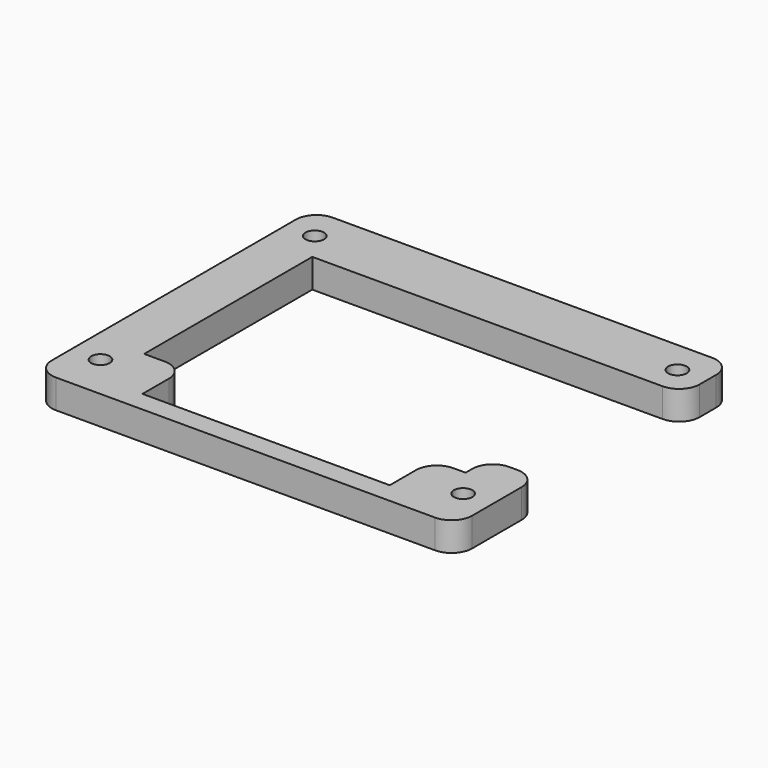
from build123d import *

# Parameters (mm, degrees)
F0_W     = 102
F0_H     = 84
F0_R     = 2.25
F0_W_2   = 78
F0_H_2   = 51
F1_DEPTH = 15
F3_DEPTH = 4
F4_W     = 12
F4_H     = 44
F4_W_2   = 60
F4_H_2   = 13
F5_DEPTH = 15.001
F6_W     = 102
F6_H     = 84
F7_DEPTH = 8
F8_R     = 5


with BuildPart() as f1:
    # F0 (on Top) → F1 (new body)
    with BuildSketch(Plane.XY):
        with Locations((0, -1.5)):
            Rectangle(F0_W, F0_H)
        with Locations((-44, -32.5)):
            Circle(F0_R, mode=Mode.SUBTRACT)
        with Locations((44, -32.5)):
            Circle(F0_R, mode=Mode.SUBTRACT)
        with Locations((-44, 32.5)):
            Circle(F0_R, mode=Mode.SUBTRACT)
        Rectangle(F0_W_2, F0_H_2, mode=Mode.SUBTRACT)
        with Locations((44, 32.5)):
            Circle(F0_R, mode=Mode.SUBTRACT)
    extrude(amount=F1_DEPTH)

    # F2 (on face) → F3 (cut)
    with BuildSketch(Plane(origin=(0, 0, 0), x_dir=(1, 0, 0), z_dir=(0, 0, -1))):
        Polygon((-41.075, 30.8112504626), (-41.075, 34.1887495374), (-44, 35.8774990748), (-46.925, 34.1887495374), (-46.925, 30.8112504626), (-44, 29.1225009252), align=None)
        Polygon((41.075, 34.1887495374), (41.075, 30.8112504626), (44, 29.1225009252), (46.925, 30.8112504626), (46.925, 34.1887495374), (44, 35.8774990748), align=None)
        Polygon((41.075, -30.8112504626), (41.075, -34.1887495374), (44, -35.8774990748), (46.925, -34.1887495374), (46.925, -30.8112504626), (44, -29.1225009252), align=None)
        Polygon((-41.075, -34.1887495374), (-41.075, -30.8112504626), (-44, -29.1225009252), (-46.925, -30.8112504626), (-46.925, -34.1887495374), (-44, -35.8774990748), align=None)
    extrude(amount=-F3_DEPTH, mode=Mode.SUBTRACT)

    # F4 (on face) → F5 (cut, through all)
    with BuildSketch(Plane.XY.offset(15)):
        with Locations((45, 3.5)):
            Rectangle(F4_W, F4_H)
        with Locations((1, -32)):
            Rectangle(F4_W_2, F4_H_2)
    extrude(amount=-F5_DEPTH, mode=Mode.SUBTRACT)

    # F6 (on face) → F7 (cut)
    with BuildSketch(Plane.XY.offset(15)):
        with Locations((0, -1.5)):
            Rectangle(F6_W, F6_H)
    extrude(amount=-F7_DEPTH, mode=Mode.SUBTRACT)

    # F8
    f8_edges = [f1.edges().sort_by_distance(p)[0] for p in [
        (-51, 40.5, 3.5),
        (51, 40.5, 3.5),
        (-51, -43.5, 3.5),
        (51, -43.5, 3.5),
        (51, 25.5, 3.5),
        (51, -18.5, 3.5),
        (39, -18.5, 3.5),
        (31, -25.5, 3.5),
        (-29, -25.5, 3.5),
    ]]
    fillet(f8_edges, radius=F8_R)


solid = f1.part
